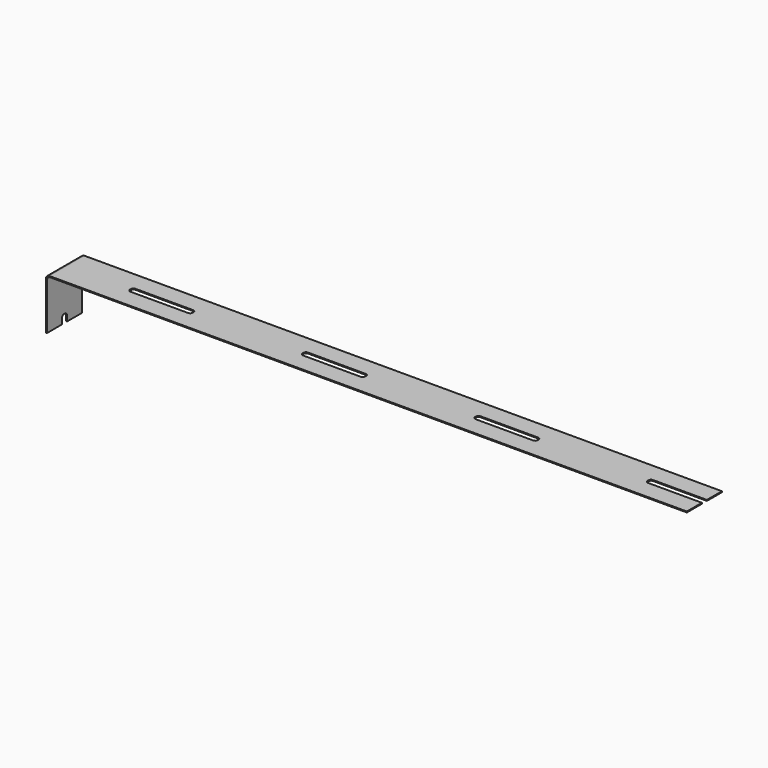
from build123d import *

# Parameters (mm, degrees)
F0_W     = 4
F0_H     = 3
F1_DEPTH = 0.15
F2_DEPTH = 1.9
F3_W     = 0.15
F3_H     = 7
F4_DEPTH = 8
F6_DEPTH = 25
F7_R     = 0.5


with BuildPart() as f1:
    # F0 (on Top) → F1 (new body)
    with BuildSketch(Plane.XY):
        with BuildLine():
            Line((0, 3.5), (0, -3.5))
            Line((0, -3.5), (13.775, -3.5))
            Line((13.775, -3.5), (13.775, -0.5))
            Line((13.775, -0.5), (9.175, -0.5))
            ThreePointArc((9.175, -0.5), (8.8921572875, -0.3828427125), (8.775, -0.1))
            Line((8.775, -0.1), (8.775, 0.1))
            ThreePointArc((8.775, 0.1), (8.8921572875, 0.3828427125), (9.175, 0.5))
            Line((9.175, 0.5), (13.775, 0.5))
            Line((13.775, 0.5), (13.775, 3.5))
            Line((13.775, 3.5), (0, 3.5))
        make_face()
        with BuildLine():
            Line((13.775, -0.5), (13.775, -3.5))
            Line((13.775, -3.5), (27.55, -3.5))
            Line((27.55, -3.5), (41.325, -3.5))
            Line((41.325, -3.5), (41.325, -0.5))
            Line((41.325, -0.5), (36.725, -0.5))
            ThreePointArc((36.725, -0.5), (36.4421572875, -0.3828427125), (36.325, -0.1))
            Line((36.325, -0.1), (36.325, 0.1))
            ThreePointArc((36.325, 0.1), (36.4421572875, 0.3828427125), (36.725, 0.5))
            Line((36.725, 0.5), (41.325, 0.5))
            Line((41.325, 0.5), (41.325, 3.5))
            Line((41.325, 3.5), (27.55, 3.5))
            Line((27.55, 3.5), (13.775, 3.5))
            Line((13.775, 3.5), (13.775, 0.5))
            Line((13.775, 0.5), (18.375, 0.5))
            ThreePointArc((18.375, 0.5), (18.6578427125, 0.3828427125), (18.775, 0.1))
            Line((18.775, 0.1), (18.775, -0.1))
            ThreePointArc((18.775, -0.1), (18.6578427125, -0.3828427125), (18.375, -0.5))
            Line((18.375, -0.5), (13.775, -0.5))
        make_face()
        with BuildLine():
            Line((41.325, -0.5), (41.325, -3.5))
            Line((41.325, -3.5), (55.1, -3.5))
            Line((55.1, -3.5), (68.875, -3.5))
            Line((68.875, -3.5), (68.875, -0.5))
            Line((68.875, -0.5), (64.275, -0.5))
            ThreePointArc((64.275, -0.5), (63.9921572875, -0.3828427125), (63.875, -0.1))
            Line((63.875, -0.1), (63.875, 0.1))
            ThreePointArc((63.875, 0.1), (63.9921572875, 0.3828427125), (64.275, 0.5))
            Line((64.275, 0.5), (68.875, 0.5))
            Line((68.875, 0.5), (68.875, 3.5))
            Line((68.875, 3.5), (55.1, 3.5))
            Line((55.1, 3.5), (41.325, 3.5))
            Line((41.325, 3.5), (41.325, 0.5))
            Line((41.325, 0.5), (45.925, 0.5))
            ThreePointArc((45.925, 0.5), (46.2078427125, 0.3828427125), (46.325, 0.1))
            Line((46.325, 0.1), (46.325, -0.1))
            ThreePointArc((46.325, -0.1), (46.2078427125, -0.3828427125), (45.925, -0.5))
            Line((45.925, -0.5), (41.325, -0.5))
        make_face()
        with BuildLine():
            Line((68.875, -0.5), (68.875, -3.5))
            Line((68.875, -3.5), (82.65, -3.5))
            Line((82.65, -3.5), (96.425, -3.5))
            Line((96.425, -3.5), (96.425, -0.5))
            Line((96.425, -0.5), (91.825, -0.5))
            ThreePointArc((91.825, -0.5), (91.5421572875, -0.3828427125), (91.425, -0.1))
            Line((91.425, -0.1), (91.425, 0.1))
            ThreePointArc((91.425, 0.1), (91.5421572875, 0.3828427125), (91.825, 0.5))
            Line((91.825, 0.5), (96.425, 0.5))
            Line((96.425, 0.5), (96.425, 3.5))
            Line((96.425, 3.5), (82.65, 3.5))
            Line((82.65, 3.5), (68.875, 3.5))
            Line((68.875, 3.5), (68.875, 0.5))
            Line((68.875, 0.5), (73.475, 0.5))
            ThreePointArc((73.475, 0.5), (73.7578427125, 0.3828427125), (73.875, 0.1))
            Line((73.875, 0.1), (73.875, -0.1))
            ThreePointArc((73.875, -0.1), (73.7578427125, -0.3828427125), (73.475, -0.5))
            Line((73.475, -0.5), (68.875, -0.5))
        make_face()
        with Locations((98.425, -2)):
            Rectangle(F0_W, F0_H)
        with Locations((98.425, 2)):
            Rectangle(F0_W, F0_H)
    extrude(amount=F1_DEPTH)

    # F2 (add): a face of the model
    f2_faces = [f1.faces().sort_by_distance(p)[0] for p in [
        (0, 0, 0.075),
    ]]
    extrude(f2_faces, amount=F2_DEPTH)

    # F3 (on face) → F4 (join)
    with BuildSketch(Plane(origin=(0, 0, 0), x_dir=(1, 0, 0), z_dir=(0, 0, -1))):
        with Locations((-1.825, 0)):
            Rectangle(F3_W, F3_H)
    extrude(amount=F4_DEPTH)

    # F5 (on face) → F6 (cut)
    with BuildSketch(Plane(origin=(-1.9, 0, 0), x_dir=(0, -1, 0), z_dir=(-1, 0, 0))):
        with BuildLine():
            ThreePointArc((0.5, -7.1), (0.3828427125, -6.8171572875), (0.1, -6.7))
            Line((0.1, -6.7), (-0.1, -6.7))
            ThreePointArc((-0.1, -6.7), (-0.3828427125, -6.8171572875), (-0.5, -7.1))
            Line((-0.5, -7.1), (-0.5, -8))
            Line((-0.5, -8), (0.5, -8))
            Line((0.5, -8), (0.5, -7.1))
        make_face()
    extrude(amount=-F6_DEPTH, mode=Mode.SUBTRACT)

    # F7
    f7_edges = [f1.edges().sort_by_distance(p)[0] for p in [
        (-1.9, 0, 0.15),
        (-1.75, 0, 0),
    ]]
    fillet(f7_edges, radius=F7_R)


solid = f1.part
